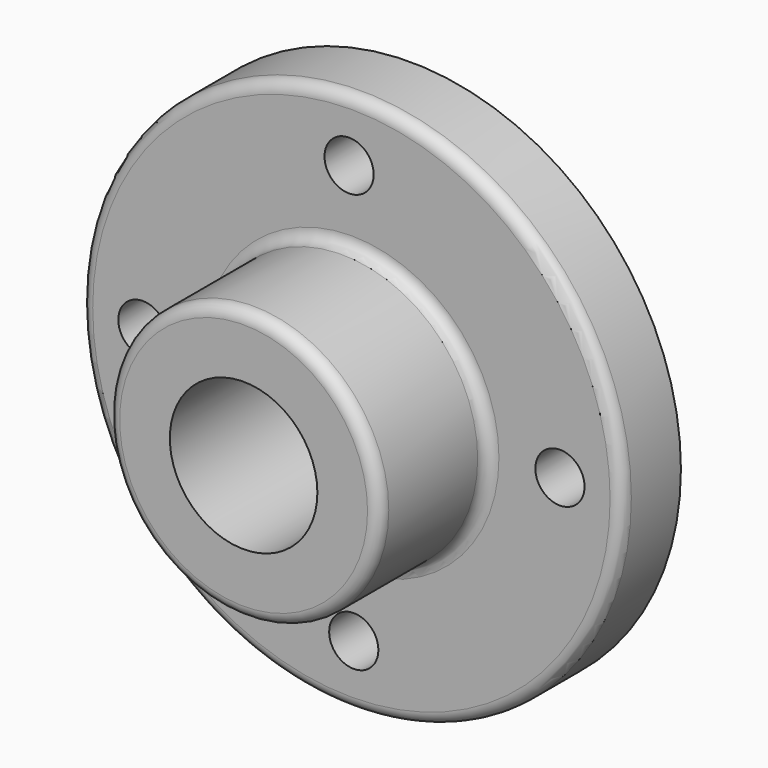
from build123d import *

# Parameters (mm, degrees)
F3_R            = 3.048
F4_R            = 3.048
F5_R            = 3.048
F2_R            = 6.35
F6_DEPTH        = 25.4
F6_COPIES_COUNT = 4


# Not quite as in the source:
# - a pattern or mirror of a feature is missing from the dataset's text; its kind, count and spacing are read off the source's solid


with BuildPart() as f1:
    # F0 (on Top) → F1 (revolve)
    with BuildSketch(Plane.XY):
        Polygon((50.8, 0), (0, 0), (0, -53.848), (16.002, -53.848), (16.002, -19.05), (50.8, -19.05), align=None)
    revolve(axis=Axis((-19.05, -27.112416923, 0), (0, -1, 0)))

    # F3
    f3_edges = [f1.edges().sort_by_distance(p)[0] for p in [
        (-88.9, -19.05, 0),
    ]]
    fillet(f3_edges, radius=F3_R)

    # F4
    f4_edges = [f1.edges().sort_by_distance(p)[0] for p in [
        (-54.102, -19.05, 0),
    ]]
    fillet(f4_edges, radius=F4_R)

    # F5
    f5_edges = [f1.edges().sort_by_distance(p)[0] for p in [
        (-54.102, -53.848, 0),
    ]]
    fillet(f5_edges, radius=F5_R)

    # F2 (on Front) → F6 (cut)
    with BuildSketch(Plane.XZ):
        with Locations((-19.6527130902, 53.848)):
            Circle(F2_R)
    f6 = extrude(amount=F6_DEPTH, mode=Mode.SUBTRACT)

    # F6_copies: F6 ×4 about axis
    f6_copies_axis = Axis((-19.05, 0, 0), (0, 1, 0))
    for i in range(1, F6_COPIES_COUNT):
        add(f6.rotate(f6_copies_axis, i * 360 / F6_COPIES_COUNT), mode=Mode.SUBTRACT)


solid = f1.part
